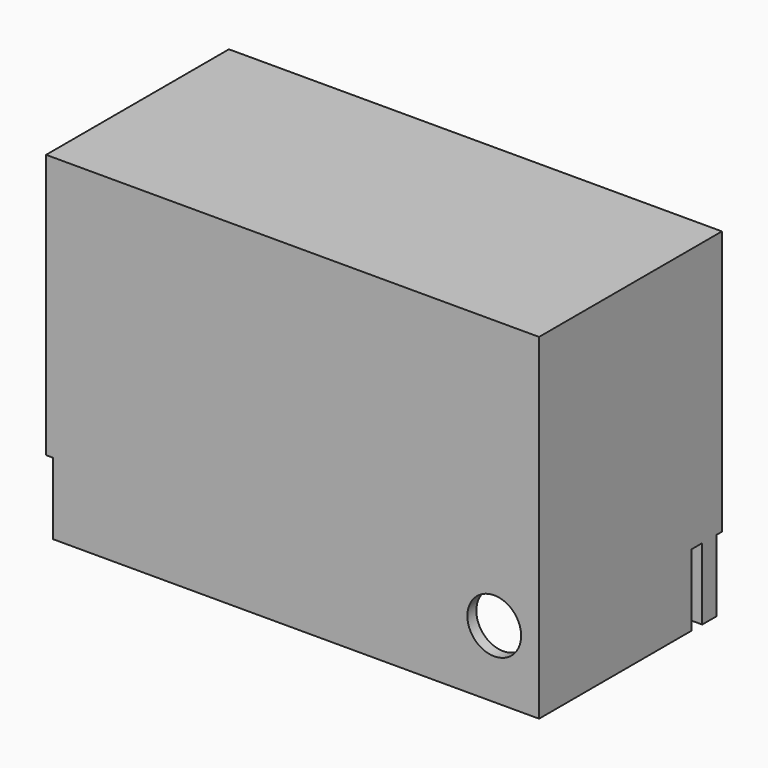
from build123d import *

# Parameters (mm, degrees)
F0_W      = 110
F0_H      = 51
F0_W_2    = 105
F0_H_2    = 46
F1_DEPTH  = 75
F3_DEPTH  = 16
F5_W      = 1
F5_H      = 3
F6_DEPTH  = 8
F8_W      = 2.5
F8_H      = 3
F9_DEPTH  = 16
F12_DEPTH = 5
F15_D     = 2
F15_DEPTH = 12
F15_TIP   = 0.600860619
F16_W     = 28
F16_H     = 47
F17_DEPTH = 12.5
F19_W     = 105
F19_H     = 46
F20_DEPTH = 1.5
F22_D     = 12
F22_DEPTH = 12
F22_TIP   = 3.6051637142
F14_R     = 1.15
F14_R_2   = 0.85
F23_DEPTH = 0.5
F25_D     = 2
F25_DEPTH = 12
F25_TIP   = 0.600860619
F24_R     = 1.15
F24_R_2   = 0.85
F26_DEPTH = 0.5


# Not quite as in the source:
# - a feature names something its author has since deleted; it is built from what else it names


with BuildPart() as f1:
    # F0 (on Top) → F1 (new body)
    with BuildSketch(Plane.XY):
        with Locations((14.1399928927, -8.9340824737)):
            Rectangle(F0_W, F0_H)
        with Locations((14.1399928927, -8.9340824737)):
            Rectangle(F0_W_2, F0_H_2, mode=Mode.SUBTRACT)
    extrude(amount=F1_DEPTH)


with BuildPart() as f3:
    # F2 (on face) → F3 (new body)
    with BuildSketch(Plane.XY):
        Polygon((-39.3600071073, -34.4340824737), (-39.3600071073, 15.0659175263), (69.1399928927, 15.0659175263), (69.1399928927, 16.5659175263), (-40.8600071073, 16.5659175263), (-40.8600071073, -34.4340824737), align=None)
    extrude(amount=F3_DEPTH)


with BuildPart() as f1_1:
    add(f1.part)

    # F4: cut F3
    add(f3.part, mode=Mode.SUBTRACT)


with BuildPart() as f6:
    # F5 (on face) → F6 (new body)
    with BuildSketch(Plane.XY):
        with Locations((-38.8600071073, 9.5659175263)):
            Rectangle(F5_W, F5_H)
    extrude(amount=F6_DEPTH)


with BuildPart() as f1_2:
    add(f1_1.part)

    # F7: cut F6
    add(f6.part, mode=Mode.SUBTRACT)


with BuildPart() as f9:
    # F8 (on face) → F9 (new body)
    with BuildSketch(Plane.XY):
        with Locations((67.8899928927, 9.5659175263)):
            Rectangle(F8_W, F8_H)
    extrude(amount=F9_DEPTH)


with BuildPart() as f1_3:
    add(f1_2.part)

    # F10: cut F9
    add(f9.part, mode=Mode.SUBTRACT)


with BuildPart() as f12:
    # F11 (on face) → F12 (new body, symmetric)
    with BuildSketch(Plane.XZ.offset(-14.0659175263)):
        with BuildLine():
            Line((62.6399928927, 0), (62.6399928927, 11))
            ThreePointArc((62.6399928927, 11), (60.1399928927, 8.5), (57.6399928927, 11))
            Line((57.6399928927, 11), (57.6399928927, 0))
            Line((57.6399928927, 0), (62.6399928927, 0))
        make_face()
        with BuildLine():
            ThreePointArc((57.6399928927, 11), (60.1399928927, 8.5), (62.6399928927, 11))
            ThreePointArc((62.6399928927, 11), (60.1399928927, 13.5), (57.6399928927, 11))
        make_face()
    extrude(amount=F12_DEPTH, both=True)


with BuildPart() as f1_4:
    add(f1_3.part)

    # F13: cut F12
    add(f12.part, mode=Mode.SUBTRACT)

    # F15
    with Locations(Plane(origin=(-39.3600071073, 0, 0), x_dir=(0, -1, 0), z_dir=(-1, 0, 0))):
        with Locations((27.9340824737, 9.5), (17.9340824737, 9.5)):
            Hole(F15_D / 2, depth=F15_DEPTH)
            with Locations((0, 0, -(F15_DEPTH + F15_TIP / 2))):  # 118° drill point
                Cone(0, F15_D / 2, F15_TIP, mode=Mode.SUBTRACT)


with BuildPart() as f17:
    # F16 (on face) → F17 (new body, symmetric)
    with BuildSketch(Plane(origin=(-40.8600071073, 0, 0), x_dir=(0, -1, 0), z_dir=(-1, 0, 0))):
        with Locations((8.9340824737, 45.5)):
            Rectangle(F16_W, F16_H)
    extrude(amount=F17_DEPTH, both=True)


with BuildPart() as f1_5:
    add(f1_4.part)

    # F18: cut F17
    add(f17.part, mode=Mode.SUBTRACT)

    # F19 (on face) → F20 (join)
    with BuildSketch(Plane.XY.offset(75)):
        with Locations((14.1399928927, -8.9340824737)):
            Rectangle(F19_W, F19_H)
    extrude(amount=-F20_DEPTH)

    # F22
    with Locations(Plane.XZ.offset(34.4340824737)):
        with Locations((59.1399928927, 15)):
            Hole(F22_D / 2, depth=F22_DEPTH)
            with Locations((0, 0, -(F22_DEPTH + F22_TIP / 2))):  # 118° drill point
                Cone(0, F22_D / 2, F22_TIP, mode=Mode.SUBTRACT)

    # F14 (on face) → F23 (join)
    with BuildSketch(Plane(origin=(-39.3600071073, 0, 0), x_dir=(0, -1, 0), z_dir=(-1, 0, 0))):
        with Locations((27.9340824737, 9.5)):
            Circle(F14_R)
        with Locations((27.9340824737, 9.5)):
            Circle(F14_R_2, mode=Mode.SUBTRACT)
        with Locations((17.9340824737, 9.5)):
            Circle(F14_R)
        with Locations((17.9340824737, 9.5)):
            Circle(F14_R_2, mode=Mode.SUBTRACT)
    extrude(amount=F23_DEPTH)

    # F25
    with Locations(Plane(origin=(0, 15.0659175263, 0), x_dir=(-1, 0, 0), z_dir=(0, 1, 0))):
        with Locations((35.8600071073, 11)):
            Hole(F25_D / 2, depth=F25_DEPTH)
            with Locations((0, 0, -(F25_DEPTH + F25_TIP / 2))):  # 118° drill point
                Cone(0, F25_D / 2, F25_TIP, mode=Mode.SUBTRACT)

    # F24 (on face) → F26 (join)
    with BuildSketch(Plane(origin=(0, 15.0659175263, 0), x_dir=(-1, 0, 0), z_dir=(0, 1, 0))):
        with Locations((35.8600071073, 11)):
            Circle(F24_R)
        with Locations((35.8600071073, 11)):
            Circle(F24_R_2, mode=Mode.SUBTRACT)
    extrude(amount=F26_DEPTH)


solid = f1_5.part
